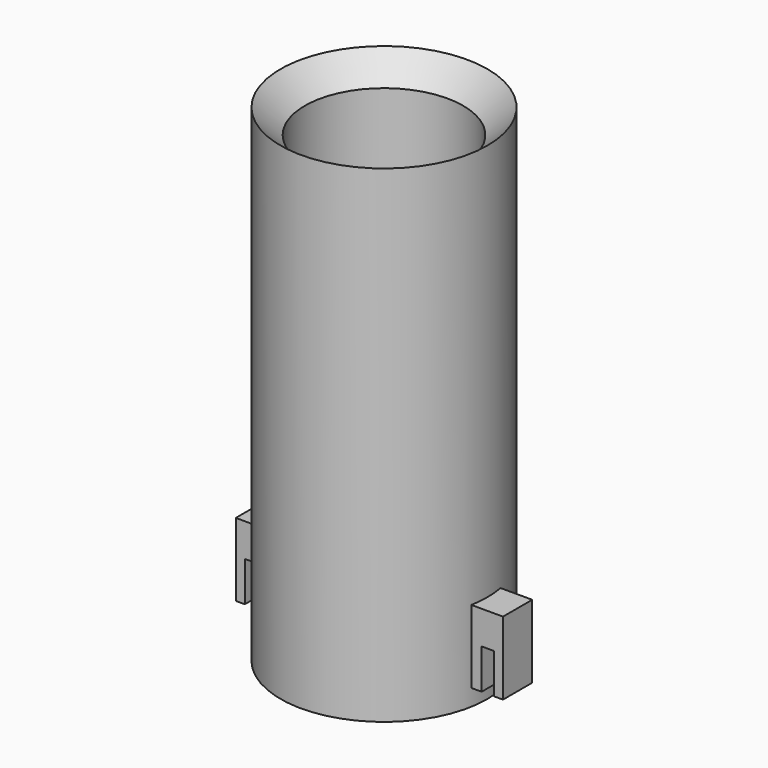
from build123d import *

# Parameters (mm, degrees)
F0_R     = 8.5
F1_DEPTH = 40
F2_T     = -2
F3_SIZE  = 1.99999
F5_DEPTH = 1.5


# Not quite as in the source:
# - a fillet or chamfer is up to 0.001 mm smaller than in the source, because OpenCascade refuses the exact size


with BuildPart() as f1:
    # F0 (on Top) → F1 (new body)
    with BuildSketch(Plane.XY):
        Circle(F0_R)
    extrude(amount=F1_DEPTH)

    # F2
    f2_openings = [f1.faces().sort_by_distance(p)[0] for p in [
        (0, 0, 40),
    ]]
    offset(amount=F2_T, openings=f2_openings)

    # F3 (size 2 in the source; OpenCascade refuses exactly that, so slightly less here)
    f3_edges = [f1.edges().sort_by_distance(p)[0] for p in [
        (-6.5, 0, 40),
    ]]
    chamfer(f3_edges, length=F3_SIZE)

    # F4 (on Front) → F5 (join, symmetric)
    with BuildSketch(Plane.XZ):
        Polygon((-8.2697293678, 1.3648961653), (-8.2697293678, 7.3648961653), (-10.9697293678, 7.3648961653), (-10.9697293678, 1.3648961653), (-10.2286748588, 1.3648961653), (-10.2286748588, 4.6420348808), (-9.2178666964, 4.6420348808), (-9.2178666964, 1.3648961653), align=None)
        Polygon((10.9697293678, 7.3648961653), (8.2697293678, 7.3648961653), (8.2697293678, 1.3648961653), (9.2178666964, 1.3648961653), (9.2178666964, 4.6420348808), (10.2286748588, 4.6420348808), (10.2286748588, 1.3648961653), (10.9697293678, 1.3648961653), align=None)
    extrude(amount=F5_DEPTH, both=True)


solid = f1.part
